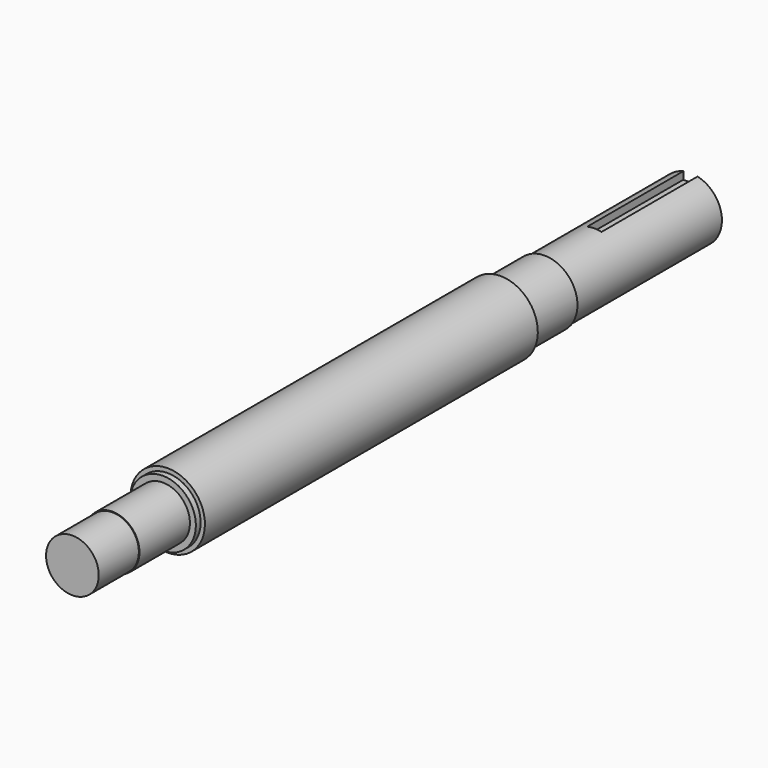
from build123d import *

# Parameters (mm, degrees)
F3_DEPTH = 66.548


# Not quite as in the source:
# - a feature names something its author has since deleted; it is built from what else it names


with BuildPart() as f1:
    # F0 (on Right) → F1 (revolve)
    with BuildSketch(Plane.YZ):
        Polygon((-107.315, 14.605), (-135.1026, 14.605), (-135.1026, 0), (0, 0), (293.1414, 0), (293.1414, 17.4625), (192.0494, 17.4625), (192.0494, 18.2626), (161.5948, 18.2626), (161.5948, 20.6375), (-69.088, 20.6375), (-69.088, 18.2626), (-72.39, 18.2626), (-72.39, 14.9606), (-107.315, 14.9606), align=None)
    revolve(axis=Axis((0, 146.5707, 0), (0, -1, 0)))

    # F2 (on face) → F3 (cut)
    with BuildSketch(Plane(origin=(0, 293.1414, 0), x_dir=(-1, 0, 0), z_dir=(0, 1, 0))):
        with BuildLine():
            Line((-3.96875, 17.0055264455), (-3.96875, 12.8397))
            Line((-3.96875, 12.8397), (3.96875, 12.8397))
            Line((3.96875, 12.8397), (3.96875, 17.0055264455))
            ThreePointArc((3.96875, 17.0055264455), (0, 17.4625), (-3.96875, 17.0055264455))
        make_face()
    extrude(amount=-F3_DEPTH, mode=Mode.SUBTRACT)


solid = f1.part
